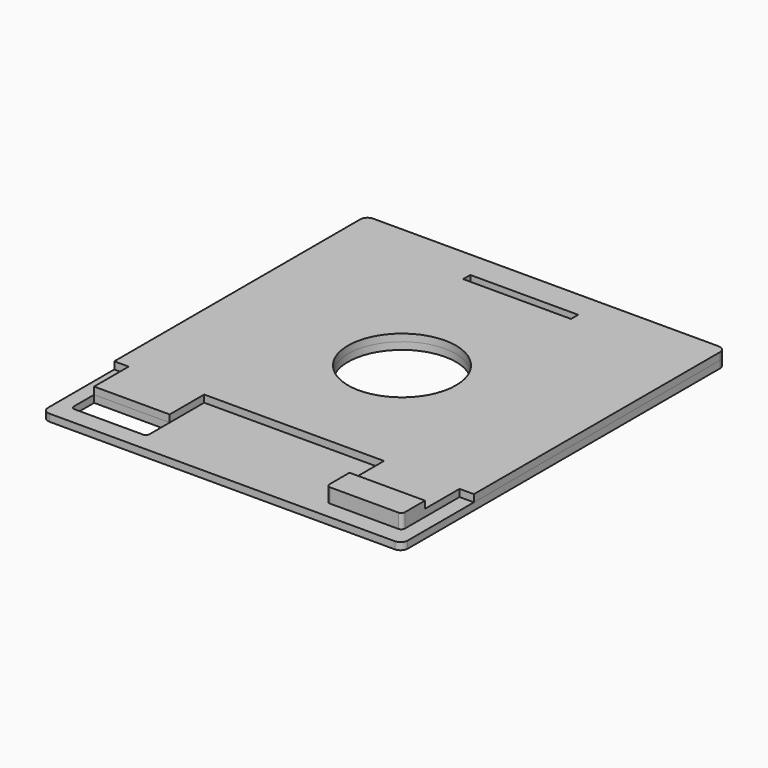
from build123d import *

# Parameters (mm, degrees)
F1_R     = 30
F2_DEPTH = 4
F3_DEPTH = 4
F4_DEPTH = 4
F5_DEPTH = 8


with BuildPart() as f2:
    # F1 (on Top) → F2 (new body)
    with BuildSketch(Plane.XY):
        with BuildLine():
            Line((249.9441257715, -40.8232776821), (57.9441257715, -40.8232776821))
            ThreePointArc((57.9441257715, -40.8232776821), (55.1156986468, -41.9948505573), (53.9441257715, -44.8232776821))
            Line((53.9441257715, -44.8232776821), (53.9441257715, -215.8232776821))
            Line((53.9441257715, -215.8232776821), (61.9441257715, -215.8232776821))
            Line((61.9441257715, -215.8232776821), (61.9441257715, -239.8232776821))
            Line((61.9441257715, -239.8232776821), (103.9441257715, -239.8232776821))
            Line((103.9441257715, -239.8232776821), (103.9441257715, -215.8232776821))
            Line((103.9441257715, -215.8232776821), (203.9441257715, -215.8232776821))
            Line((203.9441257715, -215.8232776821), (203.9441257715, -239.8232776821))
            Line((203.9441257715, -239.8232776821), (245.9441257715, -239.8232776821))
            Line((245.9441257715, -239.8232776821), (245.9441257715, -215.8232776821))
            Line((245.9441257715, -215.8232776821), (253.9441257715, -215.8232776821))
            Line((253.9441257715, -215.8232776821), (253.9441257715, -44.8232776821))
            ThreePointArc((253.9441257715, -44.8232776821), (252.7725528963, -41.9948505573), (249.9441257715, -40.8232776821))
        make_face()
        with BuildLine():
            Line((124.9441257715, -85.8232776821), (153.9441257715, -85.8232776821))
            Line((153.9441257715, -85.8232776821), (182.9441257715, -85.8232776821))
            ThreePointArc((182.9441257715, -85.8232776821), (183.6512325527, -86.1161709009), (183.9441257715, -86.8232776821))
            Line((183.9441257715, -86.8232776821), (183.9441257715, -89.8232776821))
            ThreePointArc((183.9441257715, -89.8232776821), (184.2370189903, -90.5303844633), (184.9441257715, -90.8232776821))
            Line((184.9441257715, -90.8232776821), (202.9441257715, -90.8232776821))
            ThreePointArc((202.9441257715, -90.8232776821), (203.6512325527, -91.1161709009), (203.9441257715, -91.8232776821))
            Line((203.9441257715, -91.8232776821), (203.9441257715, -140.8232776821))
            Line((203.9441257715, -140.8232776821), (203.9441257715, -189.8232776821))
            ThreePointArc((203.9441257715, -189.8232776821), (203.6512325527, -190.5303844633), (202.9441257715, -190.8232776821))
            Line((202.9441257715, -190.8232776821), (184.9441257715, -190.8232776821))
            ThreePointArc((184.9441257715, -190.8232776821), (184.2370189903, -191.1161709009), (183.9441257715, -191.8232776821))
            Line((183.9441257715, -191.8232776821), (183.9441257715, -194.8232776821))
            ThreePointArc((183.9441257715, -194.8232776821), (183.6512325527, -195.5303844633), (182.9441257715, -195.8232776821))
            Line((182.9441257715, -195.8232776821), (153.9441257715, -195.8232776821))
            Line((153.9441257715, -195.8232776821), (124.9441257715, -195.8232776821))
            ThreePointArc((124.9441257715, -195.8232776821), (124.2370189903, -195.5303844633), (123.9441257715, -194.8232776821))
            Line((123.9441257715, -194.8232776821), (123.9441257715, -191.8232776821))
            ThreePointArc((123.9441257715, -191.8232776821), (123.6512325527, -191.1161709009), (122.9441257715, -190.8232776821))
            Line((122.9441257715, -190.8232776821), (104.9441257715, -190.8232776821))
            ThreePointArc((104.9441257715, -190.8232776821), (104.2370189903, -190.5303844633), (103.9441257715, -189.8232776821))
            Line((103.9441257715, -189.8232776821), (103.9441257715, -140.8232776821))
            Line((103.9441257715, -140.8232776821), (103.9441257715, -91.8232776821))
            ThreePointArc((103.9441257715, -91.8232776821), (104.2370189903, -91.1161709009), (104.9441257715, -90.8232776821))
            Line((104.9441257715, -90.8232776821), (122.9441257715, -90.8232776821))
            ThreePointArc((122.9441257715, -90.8232776821), (123.6512325527, -90.5303844633), (123.9441257715, -89.8232776821))
            Line((123.9441257715, -89.8232776821), (123.9441257715, -86.8232776821))
            ThreePointArc((123.9441257715, -86.8232776821), (124.2370189903, -86.1161709009), (124.9441257715, -85.8232776821))
        make_face(mode=Mode.SUBTRACT)
        Polygon((123.9441257715, -60.8232776821), (123.9441257715, -55.8232776821), (153.9441257715, -55.8232776821), (183.9441257715, -55.8232776821), (183.9441257715, -60.8232776821), (153.9441257715, -60.8232776821), align=None, mode=Mode.SUBTRACT)
        with BuildLine():
            Line((245.9441257715, -253.8232776821), (245.9441257715, -239.8232776821))
            Line((245.9441257715, -239.8232776821), (203.9441257715, -239.8232776821))
            Line((203.9441257715, -239.8232776821), (203.9441257715, -253.8232776821))
            ThreePointArc((203.9441257715, -253.8232776821), (204.5299122091, -255.2374912444), (205.9441257715, -255.8232776821))
            Line((205.9441257715, -255.8232776821), (243.9441257715, -255.8232776821))
            ThreePointArc((243.9441257715, -255.8232776821), (245.3583393339, -255.2374912444), (245.9441257715, -253.8232776821))
        make_face()
        with BuildLine():
            Line((182.9441257715, -85.8232776821), (153.9441257715, -85.8232776821))
            Line((153.9441257715, -85.8232776821), (124.9441257715, -85.8232776821))
            ThreePointArc((124.9441257715, -85.8232776821), (124.2370189903, -86.1161709009), (123.9441257715, -86.8232776821))
            Line((123.9441257715, -86.8232776821), (123.9441257715, -89.8232776821))
            ThreePointArc((123.9441257715, -89.8232776821), (123.6512325527, -90.5303844633), (122.9441257715, -90.8232776821))
            Line((122.9441257715, -90.8232776821), (104.9441257715, -90.8232776821))
            ThreePointArc((104.9441257715, -90.8232776821), (104.2370189903, -91.1161709009), (103.9441257715, -91.8232776821))
            Line((103.9441257715, -91.8232776821), (103.9441257715, -140.8232776821))
            Line((103.9441257715, -140.8232776821), (103.9441257715, -189.8232776821))
            ThreePointArc((103.9441257715, -189.8232776821), (104.2370189903, -190.5303844633), (104.9441257715, -190.8232776821))
            Line((104.9441257715, -190.8232776821), (122.9441257715, -190.8232776821))
            ThreePointArc((122.9441257715, -190.8232776821), (123.6512325527, -191.1161709009), (123.9441257715, -191.8232776821))
            Line((123.9441257715, -191.8232776821), (123.9441257715, -194.8232776821))
            ThreePointArc((123.9441257715, -194.8232776821), (124.2370189903, -195.5303844633), (124.9441257715, -195.8232776821))
            Line((124.9441257715, -195.8232776821), (153.9441257715, -195.8232776821))
            Line((153.9441257715, -195.8232776821), (182.9441257715, -195.8232776821))
            ThreePointArc((182.9441257715, -195.8232776821), (183.6512325527, -195.5303844633), (183.9441257715, -194.8232776821))
            Line((183.9441257715, -194.8232776821), (183.9441257715, -191.8232776821))
            ThreePointArc((183.9441257715, -191.8232776821), (184.2370189903, -191.1161709009), (184.9441257715, -190.8232776821))
            Line((184.9441257715, -190.8232776821), (202.9441257715, -190.8232776821))
            ThreePointArc((202.9441257715, -190.8232776821), (203.6512325527, -190.5303844633), (203.9441257715, -189.8232776821))
            Line((203.9441257715, -189.8232776821), (203.9441257715, -140.8232776821))
            Line((203.9441257715, -140.8232776821), (203.9441257715, -91.8232776821))
            ThreePointArc((203.9441257715, -91.8232776821), (203.6512325527, -91.1161709009), (202.9441257715, -90.8232776821))
            Line((202.9441257715, -90.8232776821), (184.9441257715, -90.8232776821))
            ThreePointArc((184.9441257715, -90.8232776821), (184.2370189903, -90.5303844633), (183.9441257715, -89.8232776821))
            Line((183.9441257715, -89.8232776821), (183.9441257715, -86.8232776821))
            ThreePointArc((183.9441257715, -86.8232776821), (183.6512325527, -86.1161709009), (182.9441257715, -85.8232776821))
        make_face()
        with Locations((153.9441257715, -140.8232776821)):
            Circle(F1_R, mode=Mode.SUBTRACT)
    extrude(amount=F2_DEPTH)

    # F1 (on Top) → F5 (join)
    with BuildSketch(Plane.XY):
        with BuildLine():
            Line((245.9441257715, -253.8232776821), (245.9441257715, -239.8232776821))
            Line((245.9441257715, -239.8232776821), (203.9441257715, -239.8232776821))
            Line((203.9441257715, -239.8232776821), (203.9441257715, -253.8232776821))
            ThreePointArc((203.9441257715, -253.8232776821), (204.5299122091, -255.2374912444), (205.9441257715, -255.8232776821))
            Line((205.9441257715, -255.8232776821), (243.9441257715, -255.8232776821))
            ThreePointArc((243.9441257715, -255.8232776821), (245.3583393339, -255.2374912444), (245.9441257715, -253.8232776821))
        make_face()
    extrude(amount=F5_DEPTH)


with BuildPart() as f3:
    # F1 (on Top) → F3 (new body)
    with BuildSketch(Plane.XY):
        with BuildLine():
            Line((182.9441257715, -85.8232776821), (153.9441257715, -85.8232776821))
            Line((153.9441257715, -85.8232776821), (124.9441257715, -85.8232776821))
            ThreePointArc((124.9441257715, -85.8232776821), (124.2370189903, -86.1161709009), (123.9441257715, -86.8232776821))
            Line((123.9441257715, -86.8232776821), (123.9441257715, -89.8232776821))
            ThreePointArc((123.9441257715, -89.8232776821), (123.6512325527, -90.5303844633), (122.9441257715, -90.8232776821))
            Line((122.9441257715, -90.8232776821), (104.9441257715, -90.8232776821))
            ThreePointArc((104.9441257715, -90.8232776821), (104.2370189903, -91.1161709009), (103.9441257715, -91.8232776821))
            Line((103.9441257715, -91.8232776821), (103.9441257715, -140.8232776821))
            Line((103.9441257715, -140.8232776821), (103.9441257715, -189.8232776821))
            ThreePointArc((103.9441257715, -189.8232776821), (104.2370189903, -190.5303844633), (104.9441257715, -190.8232776821))
            Line((104.9441257715, -190.8232776821), (122.9441257715, -190.8232776821))
            ThreePointArc((122.9441257715, -190.8232776821), (123.6512325527, -191.1161709009), (123.9441257715, -191.8232776821))
            Line((123.9441257715, -191.8232776821), (123.9441257715, -194.8232776821))
            ThreePointArc((123.9441257715, -194.8232776821), (124.2370189903, -195.5303844633), (124.9441257715, -195.8232776821))
            Line((124.9441257715, -195.8232776821), (153.9441257715, -195.8232776821))
            Line((153.9441257715, -195.8232776821), (182.9441257715, -195.8232776821))
            ThreePointArc((182.9441257715, -195.8232776821), (183.6512325527, -195.5303844633), (183.9441257715, -194.8232776821))
            Line((183.9441257715, -194.8232776821), (183.9441257715, -191.8232776821))
            ThreePointArc((183.9441257715, -191.8232776821), (184.2370189903, -191.1161709009), (184.9441257715, -190.8232776821))
            Line((184.9441257715, -190.8232776821), (202.9441257715, -190.8232776821))
            ThreePointArc((202.9441257715, -190.8232776821), (203.6512325527, -190.5303844633), (203.9441257715, -189.8232776821))
            Line((203.9441257715, -189.8232776821), (203.9441257715, -140.8232776821))
            Line((203.9441257715, -140.8232776821), (203.9441257715, -91.8232776821))
            ThreePointArc((203.9441257715, -91.8232776821), (203.6512325527, -91.1161709009), (202.9441257715, -90.8232776821))
            Line((202.9441257715, -90.8232776821), (184.9441257715, -90.8232776821))
            ThreePointArc((184.9441257715, -90.8232776821), (184.2370189903, -90.5303844633), (183.9441257715, -89.8232776821))
            Line((183.9441257715, -89.8232776821), (183.9441257715, -86.8232776821))
            ThreePointArc((183.9441257715, -86.8232776821), (183.6512325527, -86.1161709009), (182.9441257715, -85.8232776821))
        make_face()
        with Locations((153.9441257715, -140.8232776821)):
            Circle(F1_R, mode=Mode.SUBTRACT)
    extrude(amount=-F3_DEPTH)


with BuildPart() as f4:
    # F1 (on Top) → F4 (new body)
    with BuildSketch(Plane.XY):
        with BuildLine():
            Line((61.9441257715, -215.8232776821), (53.9441257715, -215.8232776821))
            Line((53.9441257715, -215.8232776821), (53.9441257715, -261.8232776821))
            ThreePointArc((53.9441257715, -261.8232776821), (55.1156986468, -264.6517048068), (57.9441257715, -265.8232776821))
            Line((57.9441257715, -265.8232776821), (249.9441257715, -265.8232776821))
            ThreePointArc((249.9441257715, -265.8232776821), (252.7725528963, -264.6517048068), (253.9441257715, -261.8232776821))
            Line((253.9441257715, -261.8232776821), (253.9441257715, -215.8232776821))
            Line((253.9441257715, -215.8232776821), (245.9441257715, -215.8232776821))
            Line((245.9441257715, -215.8232776821), (245.9441257715, -239.8232776821))
            Line((245.9441257715, -239.8232776821), (245.9441257715, -253.8232776821))
            ThreePointArc((245.9441257715, -253.8232776821), (245.3583393339, -255.2374912444), (243.9441257715, -255.8232776821))
            Line((243.9441257715, -255.8232776821), (205.9441257715, -255.8232776821))
            ThreePointArc((205.9441257715, -255.8232776821), (204.5299122091, -255.2374912444), (203.9441257715, -253.8232776821))
            Line((203.9441257715, -253.8232776821), (203.9441257715, -239.8232776821))
            Line((203.9441257715, -239.8232776821), (203.9441257715, -215.8232776821))
            Line((203.9441257715, -215.8232776821), (103.9441257715, -215.8232776821))
            Line((103.9441257715, -215.8232776821), (103.9441257715, -239.8232776821))
            Line((103.9441257715, -239.8232776821), (103.9441257715, -253.8232776821))
            ThreePointArc((103.9441257715, -253.8232776821), (103.3583393339, -255.2374912444), (101.9441257715, -255.8232776821))
            Line((101.9441257715, -255.8232776821), (63.9441257715, -255.8232776821))
            ThreePointArc((63.9441257715, -255.8232776821), (62.5299122091, -255.2374912444), (61.9441257715, -253.8232776821))
            Line((61.9441257715, -253.8232776821), (61.9441257715, -239.8232776821))
            Line((61.9441257715, -239.8232776821), (61.9441257715, -215.8232776821))
        make_face()
        with BuildLine():
            Line((249.9441257715, -40.8232776821), (57.9441257715, -40.8232776821))
            ThreePointArc((57.9441257715, -40.8232776821), (55.1156986468, -41.9948505573), (53.9441257715, -44.8232776821))
            Line((53.9441257715, -44.8232776821), (53.9441257715, -215.8232776821))
            Line((53.9441257715, -215.8232776821), (61.9441257715, -215.8232776821))
            Line((61.9441257715, -215.8232776821), (61.9441257715, -239.8232776821))
            Line((61.9441257715, -239.8232776821), (103.9441257715, -239.8232776821))
            Line((103.9441257715, -239.8232776821), (103.9441257715, -215.8232776821))
            Line((103.9441257715, -215.8232776821), (203.9441257715, -215.8232776821))
            Line((203.9441257715, -215.8232776821), (203.9441257715, -239.8232776821))
            Line((203.9441257715, -239.8232776821), (245.9441257715, -239.8232776821))
            Line((245.9441257715, -239.8232776821), (245.9441257715, -215.8232776821))
            Line((245.9441257715, -215.8232776821), (253.9441257715, -215.8232776821))
            Line((253.9441257715, -215.8232776821), (253.9441257715, -44.8232776821))
            ThreePointArc((253.9441257715, -44.8232776821), (252.7725528963, -41.9948505573), (249.9441257715, -40.8232776821))
        make_face()
        with BuildLine():
            Line((124.9441257715, -85.8232776821), (153.9441257715, -85.8232776821))
            Line((153.9441257715, -85.8232776821), (182.9441257715, -85.8232776821))
            ThreePointArc((182.9441257715, -85.8232776821), (183.6512325527, -86.1161709009), (183.9441257715, -86.8232776821))
            Line((183.9441257715, -86.8232776821), (183.9441257715, -89.8232776821))
            ThreePointArc((183.9441257715, -89.8232776821), (184.2370189903, -90.5303844633), (184.9441257715, -90.8232776821))
            Line((184.9441257715, -90.8232776821), (202.9441257715, -90.8232776821))
            ThreePointArc((202.9441257715, -90.8232776821), (203.6512325527, -91.1161709009), (203.9441257715, -91.8232776821))
            Line((203.9441257715, -91.8232776821), (203.9441257715, -140.8232776821))
            Line((203.9441257715, -140.8232776821), (203.9441257715, -189.8232776821))
            ThreePointArc((203.9441257715, -189.8232776821), (203.6512325527, -190.5303844633), (202.9441257715, -190.8232776821))
            Line((202.9441257715, -190.8232776821), (184.9441257715, -190.8232776821))
            ThreePointArc((184.9441257715, -190.8232776821), (184.2370189903, -191.1161709009), (183.9441257715, -191.8232776821))
            Line((183.9441257715, -191.8232776821), (183.9441257715, -194.8232776821))
            ThreePointArc((183.9441257715, -194.8232776821), (183.6512325527, -195.5303844633), (182.9441257715, -195.8232776821))
            Line((182.9441257715, -195.8232776821), (153.9441257715, -195.8232776821))
            Line((153.9441257715, -195.8232776821), (124.9441257715, -195.8232776821))
            ThreePointArc((124.9441257715, -195.8232776821), (124.2370189903, -195.5303844633), (123.9441257715, -194.8232776821))
            Line((123.9441257715, -194.8232776821), (123.9441257715, -191.8232776821))
            ThreePointArc((123.9441257715, -191.8232776821), (123.6512325527, -191.1161709009), (122.9441257715, -190.8232776821))
            Line((122.9441257715, -190.8232776821), (104.9441257715, -190.8232776821))
            ThreePointArc((104.9441257715, -190.8232776821), (104.2370189903, -190.5303844633), (103.9441257715, -189.8232776821))
            Line((103.9441257715, -189.8232776821), (103.9441257715, -140.8232776821))
            Line((103.9441257715, -140.8232776821), (103.9441257715, -91.8232776821))
            ThreePointArc((103.9441257715, -91.8232776821), (104.2370189903, -91.1161709009), (104.9441257715, -90.8232776821))
            Line((104.9441257715, -90.8232776821), (122.9441257715, -90.8232776821))
            ThreePointArc((122.9441257715, -90.8232776821), (123.6512325527, -90.5303844633), (123.9441257715, -89.8232776821))
            Line((123.9441257715, -89.8232776821), (123.9441257715, -86.8232776821))
            ThreePointArc((123.9441257715, -86.8232776821), (124.2370189903, -86.1161709009), (124.9441257715, -85.8232776821))
        make_face(mode=Mode.SUBTRACT)
        Polygon((123.9441257715, -60.8232776821), (123.9441257715, -55.8232776821), (153.9441257715, -55.8232776821), (183.9441257715, -55.8232776821), (183.9441257715, -60.8232776821), (153.9441257715, -60.8232776821), align=None, mode=Mode.SUBTRACT)
    extrude(amount=-F4_DEPTH)


solid = Compound([f2.part, f3.part, f4.part])
